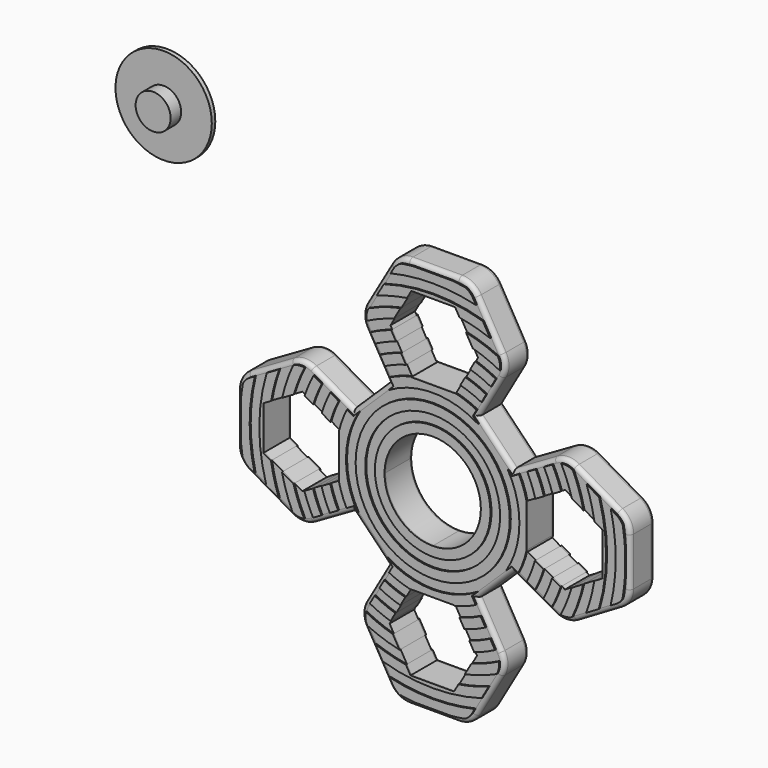
from build123d import *
from build123d import SkipClean  # not in build123d's __all__

# Parameters (mm, degrees)
F0_R          = 11.0036785857
F1_DEPTH      = 7
F2_R          = 1
F4_DEPTH      = 0.3
F4_DEPTH_BACK = 7.3
F0_R_2        = 11
F5_DEPTH      = 1
F6_R          = 8.8
F6_R_2        = 6.6
F6_R_3        = 4.4
F6_R_4        = 2.2
F7_DEPTH      = 1.3
F8_R          = 4
F9_DEPTH      = 3


with BuildPart() as f1:
    # F0 (on Front) → F1 (new body)
    with BuildSketch(Plane.XZ):
        with BuildLine():
            Line((-18.2967375063, 10.4399278195), (-27.5245304736, 15.731762043))
            ThreePointArc((-27.5245304736, 15.731762043), (-30.0191806519, 16.394354662), (-32.5118871743, 15.7244870004))
            Line((-32.5118871743, 15.7244870004), (-42.2752223977, 10.087622781))
            ThreePointArc((-42.2752223977, 10.087622781), (-44.1053494166, 8.2574957621), (-44.7752223977, 5.7574957621))
            Line((-44.7752223977, 5.7574957621), (-44.7752223977, -5.5183742625))
            ThreePointArc((-44.7752223977, -5.5183742625), (-44.1053494166, -8.0183742625), (-42.2752223977, -9.8485012815))
            Line((-42.2752223977, -9.8485012815), (-32.5100325066, -15.4864362938))
            ThreePointArc((-32.5100325066, -15.4864362938), (-30.0100325066, -16.1563092749), (-27.5100325066, -15.4864362938))
            Line((-27.5100325066, -15.4864362938), (-18.2958624745, -10.1666327454))
            Line((-18.2958624745, -10.1666327454), (-10.3889898328, -18.3056384576))
            Line((-10.3889898328, -18.3056384576), (-15.6867230324, -27.5437179393))
            ThreePointArc((-15.6867230324, -27.5437179393), (-16.3493156514, -30.0383681176), (-15.6794479898, -32.53107464))
            Line((-15.6794479898, -32.53107464), (-10.0366548741, -42.304679013))
            ThreePointArc((-10.0366548741, -42.304679013), (-8.2065278552, -44.1348060319), (-5.7065278552, -44.804679013))
            Line((-5.7065278552, -44.804679013), (5.501908517, -44.804679013))
            ThreePointArc((5.501908517, -44.804679013), (8.0040520529, -44.1335677533), (9.8345089087, -42.3003901032))
            Line((9.8345089087, -42.3003901032), (15.4879457661, -32.4859196546))
            ThreePointArc((15.4879457661, -32.4859196546), (16.1553453744, -29.9902228508), (15.4879600279, -27.4945222331))
            Line((15.4879600279, -27.4945222331), (10.2107410983, -18.3330519886))
            Line((10.2107410983, -18.3330519886), (18.2197209078, -10.5100334755))
            Line((18.2197209078, -10.5100334755), (27.5308512562, -15.768812208))
            ThreePointArc((27.5308512562, -15.768812208), (30.0369548307, -16.4149670232), (32.5303998677, -15.7215674132))
            Line((32.5303998677, -15.7215674132), (42.4107261792, -9.8923367217))
            ThreePointArc((42.4107261792, -9.8923367217), (44.2118920852, -8.0655300976), (44.8700341915, -5.5859595641))
            Line((44.8700341915, -5.5859595641), (44.8700341915, 5.4525893419))
            ThreePointArc((44.8700341915, 5.4525893419), (44.2001612104, 7.9525893419), (42.3700341915, 9.7827163608))
            Line((42.3700341915, 9.7827163608), (32.4926925689, 15.4854022054))
            ThreePointArc((32.4926925689, 15.4854022054), (29.9926925689, 16.1552751865), (27.4926925689, 15.4854022054))
            Line((27.4926925689, 15.4854022054), (18.2734107941, 10.1626473911))
            Line((18.2734107941, 10.1626473911), (10.4144589104, 18.2523254689))
            Line((10.4144589104, 18.2523254689), (15.7317619692, 27.5245304735))
            ThreePointArc((15.7317619692, 27.5245304735), (16.3943545882, 30.0191806518), (15.7244869266, 32.5118871742))
            Line((15.7244869266, 32.5118871742), (10.0876227441, 42.2752223337))
            ThreePointArc((10.0876227441, 42.2752223337), (8.2574957252, 44.1053493526), (5.7574957252, 44.7752223337))
            Line((5.7574957252, 44.7752223337), (-5.5183742256, 44.7752223337))
            ThreePointArc((-5.5183742256, 44.7752223337), (-8.0183742256, 44.1053493526), (-9.8485012445, 42.2752223337))
            Line((-9.8485012445, 42.2752223337), (-15.4880955979, 32.5071583796))
            ThreePointArc((-15.4880955979, 32.5071583796), (-16.1579679591, 30.0096481618), (-15.4905832325, 27.5114720482))
            Line((-15.4905832325, 27.5114720482), (-10.208060076, 18.3407934466))
            Line((-10.208060076, 18.3407934466), (-18.2967375063, 10.4399278195))
        make_face()
        Polygon((-30.0100325066, 10.1229049187), (-21.3468823335, 5.1548746722), (-21.3468823335, -4.8821113346), (-30.0100325066, -9.8837834191), (-38.6731826796, -4.8821113346), (-38.6731826796, 5.1212328342), align=None, mode=Mode.SUBTRACT)
        Polygon((4.9016841594, -21.3414827727), (9.8835483221, -29.9902049305), (4.8649180178, -38.7026395178), (-5.070265056, -38.7026395178), (-10.0778661652, -30.0292199726), (-5.0957360715, -21.3414827727), align=None, mode=Mode.SUBTRACT)
        Circle(F0_R, mode=Mode.SUBTRACT)
        Polygon((38.7679942454, 4.8163262823), (38.7679942454, -4.9566009246), (29.9776834671, -10.1427403052), (21.4515147548, -5.3272954541), (21.4515147548, 4.9514977573), (29.9926925689, 9.8827490675), align=None, mode=Mode.SUBTRACT)
        Polygon((5.1212328342, 38.6731826796), (10.1229049187, 30.0100325066), (5.1479964163, 21.3348881707), (-4.8907450514, 21.3348881707), (-9.8858085371, 30.0065248992), (-4.8821113346, 38.6731826796), align=None, mode=Mode.SUBTRACT)
    extrude(amount=F1_DEPTH)

    # F2
    f2_edges = [f1.edges().sort_by_distance(p)[0] for p in [
        (12.661227, -7, -37.393155),
        (-44.775222, -7, 0.119561),
        (-12.668298, -7, 37.39119),
        (22.883052, -7, 12.824025),
        (14.343935, -7, 14.207486),
        (14.343935, 0, 14.207486),
        (13.07311, 0, 22.888428),
        (37.431363, 0, 12.634059),
        (-14.252399, 0, 14.390361),
        (-22.910634, 0, 13.085845),
        (-14.342426, 0, -14.236136),
        (-13.037856, 0, -22.924678),
        (14.215231, 0, -14.421543),
        (14.215231, -7, -14.421543),
        (-14.342426, -7, -14.236136),
        (-14.252399, -7, 14.390361),
    ]]
    fillet(f2_edges, radius=F2_R)

    # F3 (on face) → F4 (join, two sides)
    with BuildSketch(Plane.XZ.offset(7)) as f4_sk:
        with BuildLine():
            ThreePointArc((-9.6128247712, 40.6834259597), (-4.8389401255, 41.5226709926), (0, 41.8036786407))
            Line((0, 41.8036786407), (0, 43.7752223337))
            Line((0, 43.7752223337), (-4.47812947, 43.7752223337))
            ThreePointArc((-4.47812947, 43.7752223337), (-5.8315398546, 43.6155577385), (-7.1793569553, 43.4140595617))
            ThreePointArc((-7.1793569553, 43.4140595617), (-8.2087402324, 42.735278203), (-8.9824758407, 41.7752223337))
            Line((-8.9824758407, 41.7752223337), (-9.6128247712, 40.6834259597))
        make_face()
        with BuildLine():
            Line((0, 43.7752223337), (0, 41.8036786407))
            ThreePointArc((0, 41.8036786407), (4.9806722623, 41.5059086362), (9.8903892952, 40.6168406881))
            Line((9.8903892952, 40.6168406881), (9.2215973403, 41.7752223337))
            ThreePointArc((9.2215973403, 41.7752223337), (8.5013230308, 42.6857913016), (7.5498931163, 43.3511573992))
            ThreePointArc((7.5498931163, 43.3511573992), (6.0177478845, 43.5902563002), (4.47812947, 43.7752223337))
            Line((4.47812947, 43.7752223337), (0, 43.7752223337))
        make_face()
        with BuildLine():
            Line((-4.8821113346, 38.6731826796), (0, 38.6731826796))
            Line((0, 38.6731826796), (0, 39.6036786407))
            ThreePointArc((0, 39.6036786407), (-5.6391555639, 39.200143959), (-11.1633927705, 37.9977634043))
            Line((-11.1633927705, 37.9977634043), (-12.8129660904, 35.1406186033))
            ThreePointArc((-12.8129660904, 35.1406186033), (-9.3915444314, 36.2054425336), (-5.8839296525, 36.9379824531))
            Line((-5.8839296525, 36.9379824531), (-4.8821113346, 38.6731826796))
        make_face()
        with BuildLine():
            Line((0, 39.6036786407), (0, 38.6731826796))
            Line((0, 38.6731826796), (5.1212328342, 38.6731826796))
            Line((5.1212328342, 38.6731826796), (6.1478854257, 36.8949682294))
            ThreePointArc((6.1478854257, 36.8949682294), (9.677525929, 36.1300521416), (13.1169411028, 35.0282890242))
            Line((13.1169411028, 35.0282890242), (11.4521899821, 37.9117225471))
            ThreePointArc((11.4521899821, 37.9117225471), (5.7882504008, 39.1784062868), (0, 39.6036786407))
        make_face()
        with BuildLine():
            ThreePointArc((-15.1028332191, 29.3453102314), (-12.0407555772, 30.7288627995), (-8.8538695838, 31.7938955967))
            Line((-8.8538695838, 31.7938955967), (-7.3307943396, 34.4319393034))
            ThreePointArc((-7.3307943396, 34.4319393034), (-11.0356824812, 33.4292192851), (-14.6093886059, 32.0291235347))
            Line((-14.6093886059, 32.0291235347), (-14.6220701941, 32.0071583796))
            ThreePointArc((-14.6220701941, 32.0071583796), (-15.0942808295, 30.7181055409), (-15.1028332191, 29.3453102314))
        make_face()
        with BuildLine():
            Line((7.6041766003, 34.3725979244), (9.1397574529, 31.7128938686))
            ThreePointArc((9.1397574529, 31.7128938686), (12.2915073837, 30.6294245793), (15.3179160239, 29.2336151118))
            ThreePointArc((15.3179160239, 29.2336151118), (15.352317709, 30.5903074739), (14.9311095602, 31.8804165145))
            ThreePointArc((14.9311095602, 31.8804165145), (11.3363363848, 33.3284633191), (7.6041766003, 34.3725979244))
        make_face()
        with BuildLine():
            ThreePointArc((-13.1278761521, 25.4131717721), (-10.7870101117, 26.4917127539), (-8.3585619797, 27.3551617326))
            Line((-8.3585619797, 27.3551617326), (-9.4832107673, 29.3075985257))
            ThreePointArc((-9.4832107673, 29.3075985257), (-11.8966530782, 28.4136633213), (-14.2270475361, 27.3213787391))
            Line((-14.2270475361, 27.3213787391), (-13.1278761521, 25.4131717721))
        make_face()
        with BuildLine():
            Line((9.6826445581, 29.2423154378), (8.5639501884, 27.2915589323))
            ThreePointArc((8.5639501884, 27.2915589323), (10.9829019117, 26.4111017828), (13.3129008316, 25.3167356353))
            Line((13.3129008316, 25.3167356353), (14.4080175007, 27.2263778256))
            ThreePointArc((14.4080175007, 27.2263778256), (12.0874315188, 28.3330304958), (9.6826445581, 29.2423154378))
        make_face()
        with BuildLine():
            ThreePointArc((-10.9289490395, 21.5957433916), (-8.5604573489, 22.6392718461), (-6.0940786549, 23.4239250573))
            Line((-6.0940786549, 23.4239250573), (-7.2292985773, 25.3947137775))
            ThreePointArc((-7.2292985773, 25.3947137775), (-9.6751762236, 24.5671571576), (-12.0285262548, 23.5046548986))
            Line((-12.0285262548, 23.5046548986), (-10.9289490395, 21.5957433916))
        make_face()
        with BuildLine():
            Line((7.4410538669, 25.3334751488), (6.3127401872, 23.3659446861))
            ThreePointArc((6.3127401872, 23.3659446861), (8.7674709204, 22.5599094281), (11.1222963372, 21.4968040399))
            Line((11.1222963372, 21.4968040399), (12.2176707679, 23.4068957098))
            ThreePointArc((12.2176707679, 23.4068957098), (9.8764513187, 24.4869343755), (7.4410538669, 25.3334751488))
        make_face()
        with BuildLine():
            ThreePointArc((-10.13637045, 17.012926903), (-5.256764717, 19.0932478226), (0, 19.8036786407))
            Line((0, 19.8036786407), (0, 21.3348881707))
            Line((0, 21.3348881707), (-4.8907450514, 21.3348881707))
            Line((-4.8907450514, 21.3348881707), (-4.9509715655, 21.4394438893))
            ThreePointArc((-4.9509715655, 21.4394438893), (-7.4418287045, 20.7070292234), (-9.8290761097, 19.686318512))
            Line((-9.8290761097, 19.686318512), (-8.9542556636, 18.1675940489))
            Line((-8.9542556636, 18.1675940489), (-10.13637045, 17.012926903))
        make_face()
        with BuildLine():
            Line((0, 21.3348881707), (0, 19.8036786407))
            ThreePointArc((0, 19.8036786407), (5.3766369365, 19.0598390066), (10.3493735953, 16.8841983491))
            Line((10.3493735953, 16.8841983491), (9.1720796265, 18.0960557763))
            Line((9.1720796265, 18.0960557763), (10.0267341505, 19.5863849651))
            ThreePointArc((10.0267341505, 19.5863849651), (7.655062429, 20.6291515321), (5.1772645799, 21.3859253995))
            Line((5.1772645799, 21.3859253995), (5.1479964163, 21.3348881707))
            Line((5.1479964163, 21.3348881707), (0, 21.3348881707))
        make_face()
        with BuildLine():
            Line((-17.6036786407, 0), (-15.4036786407, 0))
            ThreePointArc((-15.4036786407, 0), (-10.8920456221, 10.8920456221), (0, 15.4036786407))
            Line((0, 15.4036786407), (0, 17.6036786407))
            ThreePointArc((0, 17.6036786407), (-12.4476805407, 12.4476805407), (-17.6036786407, 0))
        make_face()
        with BuildLine():
            ThreePointArc((0, 15.4036786407), (10.8920456221, 10.8920456221), (15.4036786407, 0))
            Line((15.4036786407, 0), (17.6036786407, 0))
            ThreePointArc((17.6036786407, 0), (12.4476805407, 12.4476805407), (0, 17.6036786407))
            Line((0, 17.6036786407), (0, 15.4036786407))
        make_face()
        with BuildLine():
            Line((-13.2036786526, 0), (-11.0036785857, 0))
            ThreePointArc((-11.0036785857, 0), (-7.780775746, 7.780775746), (0, 11.0036785857))
            Line((0, 11.0036785857), (0, 13.2036786526))
            ThreePointArc((0, 13.2036786526), (-9.3364107119, 9.3364107119), (-13.2036786526, 0))
        make_face()
        with BuildLine():
            ThreePointArc((0, 11.0036785857), (7.780775746, 7.780775746), (11.0036785857, 0))
            Line((11.0036785857, 0), (13.2036786526, 0))
            ThreePointArc((13.2036786526, 0), (9.3364107119, 9.3364107119), (0, 13.2036786526))
            Line((0, 13.2036786526), (0, 11.0036785857))
        make_face()
        with BuildLine():
            ThreePointArc((17.176515161, 9.8566228815), (19.1356195892, 5.1003676969), (19.8036786407, 0))
            Line((19.8036786407, 0), (21.4515147548, 0))
            Line((21.4515147548, 0), (21.4515147548, 4.8984067257))
            ThreePointArc((21.4515147548, 4.8984067257), (20.716921469, 7.414245651), (19.6884057384, 9.8248945646))
            Line((19.6884057384, 9.8248945646), (18.0988784078, 8.9071805325))
            Line((18.0988784078, 8.9071805325), (17.176515161, 9.8566228815))
        make_face()
        with BuildLine():
            ThreePointArc((21.5968604624, 10.9267414133), (22.640314391, 8.557699692), (23.4247864593, 6.0907667071))
            Line((23.4247864593, 6.0907667071), (25.3950056345, 7.2282732783))
            ThreePointArc((25.3950056345, 7.2282732783), (24.5674031778, 9.6745515071), (23.5047809963, 12.0282798471))
            Line((23.5047809963, 12.0282798471), (21.5968604624, 10.9267414133))
        make_face()
        with BuildLine():
            ThreePointArc((25.4122909063, 13.1295812072), (26.4911148686, 10.7884783358), (27.3547960129, 8.3597587808))
            Line((27.3547960129, 8.3597587808), (29.3065080336, 9.4865802414))
            ThreePointArc((29.3065080336, 9.4865802414), (28.4121847679, 11.9001838017), (27.31947836, 14.2306963969))
            Line((27.31947836, 14.2306963969), (25.4122909063, 13.1295812072))
        make_face()
        with BuildLine():
            ThreePointArc((29.345449597, 15.102562424), (30.7314093916, 12.0342544692), (31.7975573285, 8.8407099127))
            Line((31.7975573285, 8.8407099127), (34.4346178219, 7.3182023269))
            ThreePointArc((34.4346178219, 7.3182023269), (33.4338164346, 11.0217470691), (32.0359568705, 14.5943981455))
            Line((32.0359568705, 14.5943981455), (31.9926925689, 14.6193768017))
            ThreePointArc((31.9926925689, 14.6193768017), (30.7109230198, 15.0902650238), (29.345449597, 15.102562424))
        make_face()
        with BuildLine():
            Line((38.7679942454, 4.8163262823), (38.7679942454, 0))
            Line((38.7679942454, 0), (39.6036786407, 0))
            ThreePointArc((39.6036786407, 0), (39.2011301934, 5.6322955744), (38.0016681949, 11.1500931064))
            Line((38.0016681949, 11.1500931064), (35.145715785, 12.7989779991))
            ThreePointArc((35.145715785, 12.7989779991), (36.208855394, 9.3783776271), (36.9399178669, 5.8717666716))
            Line((36.9399178669, 5.8717666716), (38.7679942454, 4.8163262823))
        make_face()
        with BuildLine():
            ThreePointArc((40.6864455755, 9.600036163), (41.5234309985, 4.8324140979), (41.8036786407, 0))
            Line((41.8036786407, 0), (43.8700341915, 0))
            Line((43.8700341915, 0), (43.8700341915, 3.4269277723))
            ThreePointArc((43.8700341915, 3.4269277723), (43.6708560506, 5.4018576177), (43.382816716, 7.3657957958))
            ThreePointArc((43.382816716, 7.3657957958), (42.7334258414, 8.2456142718), (41.8700341915, 8.916690957))
            Line((41.8700341915, 8.916690957), (40.6864455755, 9.600036163))
        make_face()
        with BuildLine():
            Line((43.8700341915, 0), (41.8036786407, 0))
            ThreePointArc((41.8036786407, 0), (41.5130692858, -4.9206327202), (40.6452817171, -9.7728512745))
            Line((40.6452817171, -9.7728512745), (41.9025877817, -9.0310612901))
            ThreePointArc((41.9025877817, -9.0310612901), (42.7226736006, -8.3899653418), (43.3495742633, -7.5589777821))
            ThreePointArc((43.3495742633, -7.5589777821), (43.6587160149, -5.499113551), (43.8700341915, -3.4269277723))
            Line((43.8700341915, -3.4269277723), (43.8700341915, 0))
        make_face()
        with BuildLine():
            Line((39.6036786407, 0), (38.7679942454, 0))
            Line((38.7679942454, 0), (38.7679942454, -4.9566009246))
            Line((38.7679942454, -4.9566009246), (36.9107625229, -6.0523372208))
            ThreePointArc((36.9107625229, -6.0523372208), (36.1478623496, -9.6107868258), (35.0427525789, -13.0782517009))
            Line((35.0427525789, -13.0782517009), (37.936083041, -11.3712341188))
            ThreePointArc((37.936083041, -11.3712341188), (39.1845620335, -5.7464302064), (39.6036786407, 0))
        make_face()
        with BuildLine():
            Line((34.3863616206, -7.5416924054), (31.7200908553, -9.1147484854))
            ThreePointArc((31.7200908553, -9.1147484854), (30.6294680169, -12.2913991401), (29.2216360292, -15.3407559005))
            ThreePointArc((29.2216360292, -15.3407559005), (30.5825316141, -15.3710163413), (31.8747725608, -14.9431544206))
            ThreePointArc((31.8747725608, -14.9431544206), (33.3366147913, -11.3123429977), (34.3863616206, -7.5416924054))
        make_face()
        with BuildLine():
            ThreePointArc((27.2750630178, -8.616343143), (26.3909890478, -11.0311435882), (25.2936103778, -13.3567850113))
            Line((25.2936103778, -13.3567850113), (27.2099151716, -14.4390835635))
            ThreePointArc((27.2099151716, -14.4390835635), (28.3183169922, -12.12186209), (29.2298036374, -9.7203496398))
            Line((29.2298036374, -9.7203496398), (27.2750630178, -8.616343143))
        make_face()
        with BuildLine():
            ThreePointArc((23.3433526998, -6.3957755181), (22.5299732697, -8.8441146651), (21.4606126722, -11.1919687042))
            Line((21.4606126722, -11.1919687042), (23.3771870006, -12.2744194852))
            ThreePointArc((23.3771870006, -12.2744194852), (24.4617191317, -9.9387395018), (25.3135615747, -7.5085182403))
            Line((25.3135615747, -7.5085182403), (23.3433526998, -6.3957755181))
        make_face()
        with BuildLine():
            Line((21.4515147548, 0), (19.8036786407, 0))
            ThreePointArc((19.8036786407, 0), (19.0323503931, -5.4731459161), (16.7784501705, -10.5199476035))
            Line((16.7784501705, -10.5199476035), (18.0579226312, -9.2701833407))
            Line((18.0579226312, -9.2701833407), (19.5438420609, -10.1094070658))
            ThreePointArc((19.5438420609, -10.1094070658), (20.6626099815, -7.5642859859), (21.4515147548, -4.8984067257))
            Line((21.4515147548, -4.8984067257), (21.4515147548, 0))
        make_face()
        with BuildLine():
            ThreePointArc((15.4036786407, 0), (10.8920456221, -10.8920456221), (0, -15.4036786407))
            Line((0, -15.4036786407), (0, -17.6036786407))
            ThreePointArc((0, -17.6036786407), (12.4476805407, -12.4476805407), (17.6036786407, 0))
            Line((17.6036786407, 0), (15.4036786407, 0))
        make_face()
        with BuildLine():
            ThreePointArc((11.0036785857, 0), (7.780775746, -7.780775746), (0, -11.0036785857))
            Line((0, -11.0036785857), (0, -13.2036786526))
            ThreePointArc((0, -13.2036786526), (9.3364107119, -9.3364107119), (13.2036786526, 0))
            Line((13.2036786526, 0), (11.0036785857, 0))
        make_face()
        with BuildLine():
            Line((0, -13.2036786526), (0, -11.0036785857))
            ThreePointArc((0, -11.0036785857), (-7.780775746, -7.780775746), (-11.0036785857, 0))
            Line((-11.0036785857, 0), (-13.2036786526, 0))
            ThreePointArc((-13.2036786526, 0), (-9.3364107119, -9.3364107119), (0, -13.2036786526))
        make_face()
        with BuildLine():
            Line((0, -17.6036786407), (0, -15.4036786407))
            ThreePointArc((0, -15.4036786407), (-10.8920456221, -10.8920456221), (-15.4036786407, 0))
            Line((-15.4036786407, 0), (-17.6036786407, 0))
            ThreePointArc((-17.6036786407, 0), (-12.4476805407, -12.4476805407), (0, -17.6036786407))
        make_face()
        with BuildLine():
            ThreePointArc((-17.1381062672, -9.9232555786), (-19.125679553, -5.1375158724), (-19.8036786407, 0))
            Line((-19.8036786407, 0), (-21.3468823335, 0))
            Line((-21.3468823335, 0), (-21.3468823335, -4.8821113346))
            Line((-21.3468823335, -4.8821113346), (-21.4425818342, -4.9373634671))
            ThreePointArc((-21.4425818342, -4.9373634671), (-20.7114945074, -7.4293922359), (-19.6918823234, -9.8179246426))
            Line((-19.6918823234, -9.8179246426), (-18.1213300882, -8.9111658868))
            Line((-18.1213300882, -8.9111658868), (-17.1381062672, -9.9232555786))
        make_face()
        with BuildLine():
            Line((-21.3468823335, 0), (-19.8036786407, 0))
            ThreePointArc((-19.8036786407, 0), (-19.0301895954, 5.4806543104), (-16.7701440925, 10.5331835085))
            Line((-16.7701440925, 10.5331835085), (-18.1386158092, 9.1964864722))
            Line((-18.1386158092, 9.1964864722), (-19.5863849359, 10.0267342075))
            ThreePointArc((-19.5863849359, 10.0267342075), (-20.6291515209, 7.655062459), (-21.3859253995, 5.1772645799))
            Line((-21.3859253995, 5.1772645799), (-21.3468823335, 5.1548746722))
            Line((-21.3468823335, 5.1548746722), (-21.3468823335, 0))
        make_face()
        with BuildLine():
            Line((-25.3334751488, 7.4410538669), (-23.3659446861, 6.3127401872))
            ThreePointArc((-23.3659446861, 6.3127401872), (-22.5599094165, 8.7674709503), (-21.4968040105, 11.122296394))
            Line((-21.4968040105, 11.122296394), (-23.4068956802, 12.2176708247))
            ThreePointArc((-23.4068956802, 12.2176708247), (-24.4869343636, 9.8764513484), (-25.3334751488, 7.4410538669))
        make_face()
        with BuildLine():
            Line((-29.2423154378, 9.6826445581), (-27.2915589323, 8.5639501884))
            ThreePointArc((-27.2915589323, 8.5639501884), (-26.4111017705, 10.9829019412), (-25.3167356055, 13.3129008883))
            Line((-25.3167356055, 13.3129008883), (-27.2263777956, 14.4080175573))
            ThreePointArc((-27.2263777956, 14.4080175573), (-28.3330304833, 12.0874315483), (-29.2423154378, 9.6826445581))
        make_face()
        with BuildLine():
            Line((-34.3725979244, 7.6041766003), (-31.7128938686, 9.1397574529))
            ThreePointArc((-31.7128938686, 9.1397574529), (-30.6294245652, 12.2915074187), (-29.2336150768, 15.3179160907))
            ThreePointArc((-29.2336150768, 15.3179160907), (-30.5903074305, 15.3523177892), (-31.8804164686, 14.9311096583))
            ThreePointArc((-31.8804164686, 14.9311096583), (-33.3284633016, 11.3363364361), (-34.3725979244, 7.6041766003))
        make_face()
        with BuildLine():
            Line((-39.6036786407, 0), (-38.6731826796, 0))
            Line((-38.6731826796, 0), (-38.6731826796, 5.1212328342))
            Line((-38.6731826796, 5.1212328342), (-36.8949682294, 6.1478854257))
            ThreePointArc((-36.8949682294, 6.1478854257), (-36.1300521285, 9.6775259776), (-35.0282889889, 13.116941197))
            Line((-35.0282889889, 13.116941197), (-37.9117225201, 11.4521900716))
            ThreePointArc((-37.9117225201, 11.4521900716), (-39.17840628, 5.788250447), (-39.6036786407, 0))
        make_face()
        with BuildLine():
            Line((-43.7752223977, 0), (-41.8036786407, 0))
            ThreePointArc((-41.8036786407, 0), (-41.5059086309, 4.9806723062), (-40.6168406672, 9.8903893812))
            Line((-40.6168406672, 9.8903893812), (-41.7752223977, 9.2215973773))
            ThreePointArc((-41.7752223977, 9.2215973773), (-42.685791283, 8.5013231554), (-43.3511573553, 7.5498933684))
            ThreePointArc((-43.3511573553, 7.5498933684), (-43.5902563257, 6.0177476999), (-43.7752223977, 4.4781288447))
            Line((-43.7752223977, 4.4781288447), (-43.7752223977, 0))
        make_face()
        with BuildLine():
            ThreePointArc((-40.6834259394, -9.6128248567), (-41.5226709875, -4.8389401691), (-41.8036786407, 0))
            Line((-41.8036786407, 0), (-43.7752223977, 0))
            Line((-43.7752223977, 0), (-43.7752223977, -4.4781288447))
            ThreePointArc((-43.7752223977, -4.4781288447), (-43.6155577615, -5.8315396826), (-43.4140595157, -7.179357233))
            ThreePointArc((-43.4140595158, -7.179357233), (-42.735278178, -8.2087403672), (-41.7752223977, -8.9824758777))
            Line((-41.7752223977, -8.9824758777), (-40.6834259394, -9.6128248567))
        make_face()
        with BuildLine():
            Line((-38.6731826796, -4.8821113346), (-38.6731826796, 0))
            Line((-38.6731826796, 0), (-39.6036786407, 0))
            ThreePointArc((-39.6036786407, 0), (-39.2001439524, -5.6391556098), (-37.9977633782, -11.1633928594))
            Line((-37.9977633782, -11.1633928594), (-35.1406185692, -12.812966184))
            ThreePointArc((-35.1406185692, -12.812966184), (-36.2054425211, -9.3915444796), (-36.9379824531, -5.8839296525))
            Line((-36.9379824531, -5.8839296525), (-38.6731826796, -4.8821113346))
        make_face()
        with BuildLine():
            ThreePointArc((-29.3463249127, -15.1008614966), (-30.7292672866, -12.0397232462), (-31.7938955967, -8.8538695838))
            Line((-31.7938955967, -8.8538695838), (-34.4319393034, -7.3307943396))
            ThreePointArc((-34.4319393034, -7.3307943396), (-33.4292192679, -11.0356825335), (-32.029123489, -14.6093887062))
            Line((-32.029123489, -14.6093887062), (-32.0100325066, -14.62041089))
            ThreePointArc((-32.0100325066, -14.62041089), (-30.7200519042, -15.0927889782), (-29.3463249127, -15.1008614966))
        make_face()
        with BuildLine():
            Line((-27.3230725195, -14.2237943565), (-25.4158624785, -13.122666126))
            ThreePointArc((-25.4158624785, -13.122666126), (-26.4940863698, -10.7811789342), (-27.3571269501, -8.3521276819))
            Line((-27.3571269501, -8.3521276819), (-29.3089553993, -9.4790163625))
            ThreePointArc((-29.3089553993, -9.4790163625), (-28.4152226122, -11.8929282222), (-27.3230725195, -14.2237943565))
        make_face()
        with BuildLine():
            Line((-23.5083262037, -12.0213495442), (-21.6003744918, -10.9197931097))
            ThreePointArc((-21.6003744918, -10.9197931097), (-22.6431154714, -8.5502854626), (-23.4268147018, -6.0829608473))
            Line((-23.4268147018, -6.0829608473), (-25.3971990382, -7.2205627744))
            ThreePointArc((-25.3971990382, -7.2205627744), (-24.5702968683, -9.6672000892), (-23.5083262037, -12.0213495442))
        make_face()
        with BuildLine():
            Line((0, -21.3414827727), (0, -19.8036786407))
            ThreePointArc((0, -19.8036786407), (-5.4136374394, -19.0493626502), (-10.4148673296, -16.843878004))
            Line((-10.4148673296, -16.843878004), (-9.1466105489, -18.149368765))
            Line((-9.1466105489, -18.149368765), (-9.9833836247, -19.6085166478))
            ThreePointArc((-9.9833836247, -19.6085166478), (-7.6084841981, -20.6463759999), (-5.1280240727, -21.397785933))
            Line((-5.1280240727, -21.397785933), (-5.0957360715, -21.3414827727))
            Line((-5.0957360715, -21.3414827727), (0, -21.3414827727))
        make_face()
        with BuildLine():
            ThreePointArc((10.1229430987, -17.0209197967), (5.2492314619, -19.0953202844), (0, -19.8036786407))
            Line((0, -19.8036786407), (0, -21.3414827727))
            Line((0, -21.3414827727), (4.9016841594, -21.3414827727))
            Line((4.9016841594, -21.3414827727), (4.9572732221, -21.4379876837))
            ThreePointArc((4.9572732221, -21.4379876837), (7.4477881367, -20.7048865149), (9.8346210942, -19.6835490108))
            Line((9.8346210942, -19.6835490108), (8.956936686, -18.1598525909))
            Line((8.956936686, -18.1598525909), (10.1229430987, -17.0209197967))
        make_face()
        with BuildLine():
            ThreePointArc((10.9344772827, -21.5929448269), (8.5663557404, -22.637040643), (6.1002880655, -23.422308709))
            Line((6.1002880655, -23.422308709), (7.2354327024, -25.3929667304))
            ThreePointArc((7.2354327024, -25.3929667304), (9.6810251238, -24.5648529064), (12.0340405579, -23.5018321331))
            Line((12.0340405579, -23.5018321331), (10.9344772827, -21.5929448269))
        make_face()
        with BuildLine():
            ThreePointArc((13.1333786667, -25.4103285413), (10.7928180244, -26.4893471206), (8.3646334016, -27.3533058302))
            Line((8.3646334016, -27.3533058302), (9.4892291009, -29.3056504598))
            ThreePointArc((9.4892291009, -29.3056504598), (11.9024264592, -28.4112453473), (14.232539951, -27.3185179749))
            Line((14.232539951, -27.3185179749), (13.1333786667, -25.4103285413))
        make_face()
        with BuildLine():
            ThreePointArc((15.1030021472, -29.3452232904), (12.03549042, -30.7309253712), (8.8427911036, -31.7969786193))
            Line((8.8427911036, -31.7969786193), (7.3241593682, -34.4333512657))
            ThreePointArc((7.3241593682, -34.4333512657), (11.0237184439, -33.4331664894), (14.592633879, -32.0367605465))
            Line((14.592633879, -32.0367605465), (14.6214256878, -31.9867774366))
            ThreePointArc((14.6214256878, -31.9867774366), (15.0904853303, -30.7076160687), (15.1030021472, -29.3452232904))
        make_face()
        with BuildLine():
            ThreePointArc((9.6117411648, -40.6836819828), (4.8383871469, -41.5227354315), (0, -41.8036786407))
            Line((0, -41.8036786407), (0, -43.804679013))
            Line((0, -43.804679013), (4.1801711069, -43.804679013))
            ThreePointArc((4.1801711069, -43.804679013), (5.7188811664, -43.6304725177), (7.2505088654, -43.4022332963))
            ThreePointArc((7.2505088654, -43.4022332963), (8.2293637728, -42.730595592), (8.9679888303, -41.8012478852))
            Line((8.9679888303, -41.8012478852), (9.6117411648, -40.6836819828))
        make_face()
        with BuildLine():
            Line((4.8649180178, -38.7026395178), (0, -38.7026395178))
            Line((0, -38.7026395178), (0, -39.6036786407))
            ThreePointArc((0, -39.6036786407), (5.6363742026, -39.2005439723), (11.1580005877, -37.9993471623))
            Line((11.1580005877, -37.9993471623), (12.8025240062, -35.1444242367))
            ThreePointArc((12.8025240062, -35.1444242367), (9.3848083294, -36.2071891823), (5.8811607611, -36.9384234092))
            Line((5.8811607611, -36.9384234092), (4.8649180178, -38.7026395178))
        make_face()
        with BuildLine():
            Line((0, -43.804679013), (0, -41.8036786407))
            ThreePointArc((0, -41.8036786407), (-4.960490259, -41.5083254816), (-9.8508863772, -40.6264394881))
            Line((-9.8508863772, -40.6264394881), (-9.1706294703, -41.804679013))
            ThreePointArc((-9.1706294703, -41.804679013), (-8.4751555992, -42.6916671347), (-7.5598471768, -43.3494226557))
            ThreePointArc((-7.5598471768, -43.3494226557), (-5.8744209853, -43.6098029347), (-4.1801711069, -43.804679013))
            Line((-4.1801711069, -43.804679013), (0, -43.804679013))
        make_face()
        with BuildLine():
            Line((0, -39.6036786407), (0, -38.7026395178))
            Line((0, -38.7026395178), (-5.070265056, -38.7026395178))
            Line((-5.070265056, -38.7026395178), (-6.1103221253, -36.901207831))
            ThreePointArc((-6.1103221253, -36.901207831), (-9.6368000952, -36.1409360668), (-13.0736349331, -35.0444752492))
            Line((-13.0736349331, -35.0444752492), (-11.4110718435, -37.9241189912))
            ThreePointArc((-11.4110718435, -37.9241189912), (-5.7670070495, -39.1815389127), (0, -39.6036786407))
        make_face()
        with BuildLine():
            Line((-7.3930664863, -25.3475208589), (-6.2641891734, -23.379007544))
            ThreePointArc((-6.2641891734, -23.379007544), (-8.7213419625, -22.5777823117), (-11.079053055, -21.5191227318))
            Line((-11.079053055, -21.5191227318), (-12.1745168095, -23.4293701626))
            ThreePointArc((-12.1745168095, -23.4293701626), (-9.83068688, -24.5053431159), (-7.3930664863, -25.3475208589))
        make_face()
        with BuildLine():
            Line((-9.6355254871, -29.2578752884), (-8.5164328113, -27.3064242249))
            ThreePointArc((-8.5164328113, -27.3064242249), (-10.9374394897, -26.429961203), (-13.2698224252, -25.3393418341))
            Line((-13.2698224252, -25.3393418341), (-14.3650038332, -27.2490969148))
            ThreePointArc((-14.3650038332, -27.2490969148), (-12.0422236132, -28.3522744811), (-9.6355254871, -29.2578752884))
        make_face()
        with BuildLine():
            Line((-7.5652581827, -34.3811846577), (-9.0990373387, -31.724601232))
            ThreePointArc((-9.0990373387, -31.724601232), (-12.2486593542, -30.6465846033), (-15.2736603338, -29.2567616771))
            ThreePointArc((-15.2736603338, -29.2567616771), (-15.3067827434, -30.6128790046), (-14.8847596265, -31.9020833285))
            ThreePointArc((-14.8847596265, -31.9020833285), (-11.2932418179, -33.3430904249), (-7.5652581827, -34.3811846577))
        make_face()
    with SkipClean():  # cleaning this boolean's faces spoils the solid; the shape is the same uncleaned
        extrude(amount=F4_DEPTH)
        extrude(f4_sk.sketch, amount=-F4_DEPTH_BACK)


with BuildPart() as f5:
    # F0 (on Front) → F5 (new body)
    with BuildSketch(Plane.XZ):
        with Locations((-66.4918273687, 53.350225091)):
            Circle(F0_R_2)
    extrude(amount=F5_DEPTH)

    # F6 (on face) → F7 (join)
    with BuildSketch(Plane.XZ.offset(1)):
        with Locations((-66.4918273687, 53.350225091)):
            Circle(F6_R)
        with Locations((-66.4918273687, 53.350225091)):
            Circle(F6_R_2, mode=Mode.SUBTRACT)
        with Locations((-66.4918273687, 53.350225091)):
            Circle(F6_R_3)
        with Locations((-66.4918273687, 53.350225091)):
            Circle(F6_R_4, mode=Mode.SUBTRACT)
    extrude(amount=-F7_DEPTH)

    # F8 (on face) → F9 (join)
    with BuildSketch(Plane.XZ.offset(1)):
        with Locations((-66.4918273687, 53.350225091)):
            Circle(F8_R)
    extrude(amount=F9_DEPTH)


solid = Compound([f1.part, f5.part])
